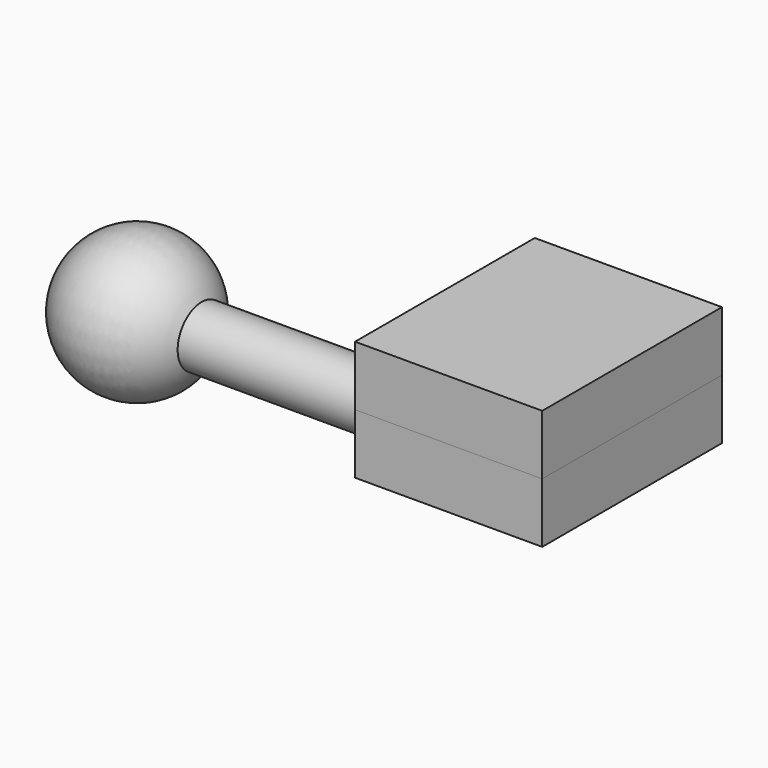
from build123d import *

# Parameters (mm, degrees)
F3_DEPTH  = 8
F4_R      = 3.55
F5_DEPTH  = 2.9
F4_R_2    = 2.5
F6_DEPTH  = 6
F7_SIZE   = 2
F8_W      = 25
F8_H      = 30
F8_R      = 2.8
F8_R_2    = 3.55
F8_R_3    = 2.5
F9_DEPTH  = 8
F10_DEPTH = 3
F11_DEPTH = 6.5


with BuildPart() as f1:
    # F0 (on Top) → F1 (revolve)
    with BuildSketch(Plane.XY):
        with BuildLine():
            Line((53.6170000059, 3.9996638481), (8.6170000059, 3.9996638481))
            ThreePointArc((8.6170000059, 3.9996638481), (-2.0481509331, 9.2765876137), (-9.4999999941, -0.0003361519))
            Line((-9.4999999941, -0.0003361519), (53.6170000059, -0.0003361519))
            Line((53.6170000059, -0.0003361519), (53.6170000059, 3.9996638481))
        make_face()
    revolve(axis=Axis((22.0585000059, -0.0003361519, 0), (-1, 0, 0)))

    # F2 (on Top) → F3 (join)
    with BuildSketch(Plane.XY):
        Polygon((66.1170000059, -15), (66.1170000059, 15), (41.1170000059, 15), (41.1170000059, 3.9996638481), (41.1170000059, -4.0003361519), (41.1170000059, -15), align=None)
    extrude(amount=F3_DEPTH)

    # F4 (on face) → F5 (cut)
    with BuildSketch(Plane.XY.offset(8)):
        with Locations((53.6170000059, 7.5)):
            Circle(F4_R)
        with Locations((47.3670000059, 0)):
            Circle(F4_R)
        with Locations((59.8670000059, 0)):
            Circle(F4_R)
        with Locations((53.6170000059, -7.5)):
            Circle(F4_R)
    extrude(amount=-F5_DEPTH, mode=Mode.SUBTRACT)

    # F4 (on face) → F6 (join)
    with BuildSketch(Plane.XY.offset(8)):
        with Locations((46.0667474743, 10.0502525317)):
            Circle(F4_R_2)
        with Locations((61.1672525376, 10.0502525317)):
            Circle(F4_R_2)
        with Locations((61.1672525376, -10.0502525317)):
            Circle(F4_R_2)
        with Locations((46.0667474743, -10.0502525317)):
            Circle(F4_R_2)
    extrude(amount=F6_DEPTH)

    # F7
    f7_edges = [f1.edges().sort_by_distance(p)[0] for p in [
        (43.566747, 10.050253, 14),
        (58.667253, 10.050253, 14),
        (58.667253, -10.050253, 14),
        (43.566747, -10.050253, 14),
    ]]
    chamfer(f7_edges, length=F7_SIZE)


with BuildPart() as f9:
    # F8 (on face) → F9 (new body)
    with BuildSketch(Plane.XY.offset(8)):
        with Locations((53.6170000059, 0)):
            Rectangle(F8_W, F8_H)
        with Locations((46.0667474743, -10.0502525317)):
            Circle(F8_R, mode=Mode.SUBTRACT)
        with Locations((61.1672525376, -10.0502525317)):
            Circle(F8_R, mode=Mode.SUBTRACT)
        with Locations((53.6170000059, -7.5)):
            Circle(F8_R_2, mode=Mode.SUBTRACT)
        with Locations((47.3670000059, 0)):
            Circle(F8_R_2, mode=Mode.SUBTRACT)
        with Locations((46.0667474743, 10.0502525317)):
            Circle(F8_R, mode=Mode.SUBTRACT)
        with Locations((59.8670000059, 0)):
            Circle(F8_R_2, mode=Mode.SUBTRACT)
        with Locations((53.6170000059, 7.5)):
            Circle(F8_R_2, mode=Mode.SUBTRACT)
        with Locations((61.1672525376, 10.0502525317)):
            Circle(F8_R, mode=Mode.SUBTRACT)
        with Locations((53.6170000059, 7.5)):
            Circle(F8_R_2)
        with Locations((59.8670000059, 0)):
            Circle(F8_R_2)
        with Locations((53.6170000059, -7.5)):
            Circle(F8_R_2)
        with Locations((47.3670000059, 0)):
            Circle(F8_R_2)
        with Locations((46.0667474743, 10.0502525317)):
            Circle(F8_R)
        with Locations((46.0667474743, 10.0502525317)):
            Circle(F8_R_3, mode=Mode.SUBTRACT)
        with Locations((61.1672525376, 10.0502525317)):
            Circle(F8_R)
        with Locations((61.1672525376, 10.0502525317)):
            Circle(F8_R_3, mode=Mode.SUBTRACT)
        with Locations((61.1672525376, -10.0502525317)):
            Circle(F8_R)
        with Locations((61.1672525376, -10.0502525317)):
            Circle(F8_R_3, mode=Mode.SUBTRACT)
        with Locations((46.0667474743, -10.0502525317)):
            Circle(F8_R)
        with Locations((46.0667474743, -10.0502525317)):
            Circle(F8_R_3, mode=Mode.SUBTRACT)
        with Locations((46.0667474743, 10.0502525317)):
            Circle(F8_R_3)
        with Locations((61.1672525376, 10.0502525317)):
            Circle(F8_R_3)
        with Locations((61.1672525376, -10.0502525317)):
            Circle(F8_R_3)
        with Locations((46.0667474743, -10.0502525317)):
            Circle(F8_R_3)
    extrude(amount=F9_DEPTH)

    # F8 (on face) → F10 (cut)
    with BuildSketch(Plane.XY.offset(8)):
        with Locations((53.6170000059, 7.5)):
            Circle(F8_R_2)
        with Locations((59.8670000059, 0)):
            Circle(F8_R_2)
        with Locations((47.3670000059, 0)):
            Circle(F8_R_2)
        with Locations((53.6170000059, -7.5)):
            Circle(F8_R_2)
    extrude(amount=F10_DEPTH, mode=Mode.SUBTRACT)

    # F8 (on face) → F11 (cut)
    with BuildSketch(Plane.XY.offset(8)):
        with Locations((46.0667474743, 10.0502525317)):
            Circle(F8_R)
        with Locations((46.0667474743, 10.0502525317)):
            Circle(F8_R_3, mode=Mode.SUBTRACT)
        with Locations((61.1672525376, 10.0502525317)):
            Circle(F8_R)
        with Locations((61.1672525376, 10.0502525317)):
            Circle(F8_R_3, mode=Mode.SUBTRACT)
        with Locations((46.0667474743, -10.0502525317)):
            Circle(F8_R)
        with Locations((46.0667474743, -10.0502525317)):
            Circle(F8_R_3, mode=Mode.SUBTRACT)
        with Locations((61.1672525376, -10.0502525317)):
            Circle(F8_R)
        with Locations((61.1672525376, -10.0502525317)):
            Circle(F8_R_3, mode=Mode.SUBTRACT)
        with Locations((46.0667474743, -10.0502525317)):
            Circle(F8_R_3)
        with Locations((46.0667474743, 10.0502525317)):
            Circle(F8_R_3)
        with Locations((61.1672525376, 10.0502525317)):
            Circle(F8_R_3)
        with Locations((61.1672525376, -10.0502525317)):
            Circle(F8_R_3)
    extrude(amount=F11_DEPTH, mode=Mode.SUBTRACT)


solid = Compound([f1.part, f9.part])
